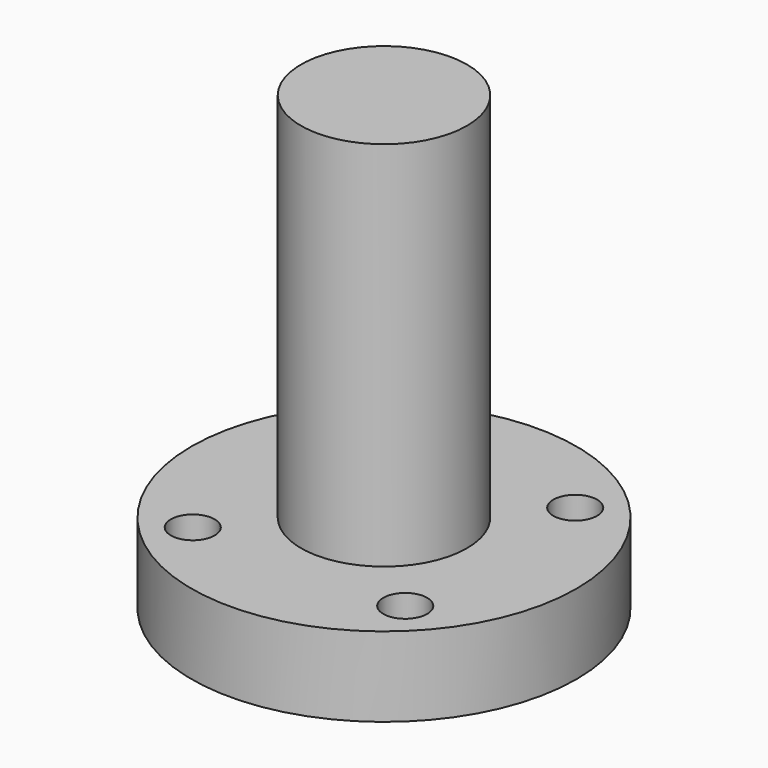
from build123d import *

# Parameters (mm, degrees)
F0_R     = 14.5
F0_R_2   = 6.25
F1_DEPTH = 6
F2_DEPTH = 28
F4_D     = 3.3
F5_D     = 11.5
F5_DEPTH = 26
F5_TIP   = 3.4549485594


with BuildPart() as f1:
    # F0 (on Top) → F1 (new body)
    with BuildSketch(Plane.XY):
        Circle(F0_R)
        Circle(F0_R_2, mode=Mode.SUBTRACT)
        Circle(F0_R_2)
    extrude(amount=-F1_DEPTH)

    # F0 (on Top) → F2 (join)
    with BuildSketch(Plane.XY):
        Circle(F0_R_2)
    extrude(amount=F2_DEPTH)

    # F4 (through all)
    with Locations(Plane(origin=(0, 0, -6), x_dir=(1, 0, 0), z_dir=(0, 0, -1))):
        with Locations((8, 8), (8, -8), (-8, -8), (-8, 8)):
            Hole(F4_D / 2)

    # F5
    with Locations(Plane(origin=(0, 0, -6), x_dir=(1, 0, 0), z_dir=(0, 0, -1))):
        with Locations((0, 0)):
            Hole(F5_D / 2, depth=F5_DEPTH)
            with Locations((0, 0, -(F5_DEPTH + F5_TIP / 2))):  # 118° drill point
                Cone(0, F5_D / 2, F5_TIP, mode=Mode.SUBTRACT)


solid = f1.part
